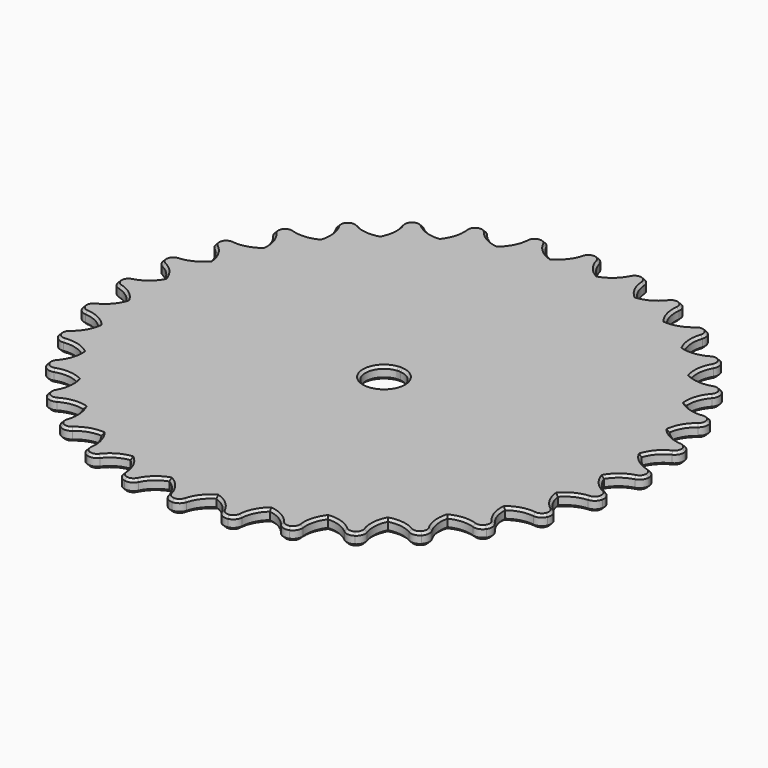
from build123d import *

# Parameters (mm, degrees)
F1_DEPTH    = 3.175
F2_C1_SIZE  = 0.635
F2_C2_SIZE  = 0.635
F2_C3_SIZE  = 0.635
F2_C4_SIZE  = 0.635
F2_C5_SIZE  = 0.635
F2_C6_SIZE  = 0.635
F2_C7_SIZE  = 0.635
F2_C8_SIZE  = 0.635
F2_C9_SIZE  = 0.635
F2_C10_SIZE = 0.635
F2_C11_SIZE = 0.635
F2_C12_SIZE = 0.635
F2_C13_SIZE = 0.635
F2_C14_SIZE = 0.635
F2_C15_SIZE = 0.635
F2_C16_SIZE = 0.635
F2_C17_SIZE = 0.635
F2_C18_SIZE = 0.635
F2_C19_SIZE = 0.635
F2_C20_SIZE = 0.635
F2_C21_SIZE = 0.635
F2_C22_SIZE = 0.635
F2_C23_SIZE = 0.635
F2_C24_SIZE = 0.635
F2_C25_SIZE = 0.635
F2_C26_SIZE = 0.635
F2_C27_SIZE = 0.635
F2_C28_SIZE = 0.635
F2_C29_SIZE = 0.635
F2_C30_SIZE = 0.635
F2_C31_SIZE = 0.635
F2_C32_SIZE = 0.635
F2_C33_SIZE = 0.635
F2_C34_SIZE = 0.635
F2_C35_SIZE = 0.635
F2_C36_SIZE = 0.635
F2_C37_SIZE = 0.635
F2_C38_SIZE = 0.635
F2_C39_SIZE = 0.635
F2_C40_SIZE = 0.635
F2_C41_SIZE = 0.635
F2_C42_SIZE = 0.635
F2_C43_SIZE = 0.635
F2_C44_SIZE = 0.635
F2_C45_SIZE = 0.635
F2_C46_SIZE = 0.635
F2_C47_SIZE = 0.635
F2_C48_SIZE = 0.635
F2_C49_SIZE = 0.635
F2_C50_SIZE = 0.635
F2_C51_SIZE = 0.635
F2_C52_SIZE = 0.635
F2_C53_SIZE = 0.635
F2_C54_SIZE = 0.635
F2_C55_SIZE = 0.635
F2_C56_SIZE = 0.635
F2_C57_SIZE = 0.635
F2_C58_SIZE = 0.635
F2_C59_SIZE = 0.635
F2_C60_SIZE = 0.635
F2_C61_SIZE = 0.635
F2_C62_SIZE = 0.635
F2_C63_SIZE = 0.635
F2_C64_SIZE = 0.635
F2_C65_SIZE = 0.635
F2_C66_SIZE = 0.635


with BuildPart() as f1:
    # F0 (on Top) → F1 (new body)
    with BuildSketch(Plane.XY):
        with BuildLine():
            ThreePointArc((66.1962592173, -2.3001108739), (67.4691190077, -1.4496131528), (67.9611963661, 0))
            ThreePointArc((67.9611963661, 0), (67.4691190077, 1.4496131528), (66.1962592173, 2.3001108739))
            ThreePointArc((66.1962592173, 2.3001108739), (63.3844227667, 3.6851664557), (61.3145216156, 6.0389532801))
            ThreePointArc((61.3145216156, 6.0389532801), (62.8854491669, 8.7513304327), (65.3730460291, 10.6583346386))
            ThreePointArc((65.3730460291, 10.6583346386), (66.4555243163, 11.7408129411), (66.6553410213, 13.25857175))
            ThreePointArc((66.6553410213, 13.25857175), (65.8899132823, 14.5843314182), (64.475587287, 15.1701644153))
            ThreePointArc((64.475587287, 15.1701644153), (61.4475685459, 15.980044464), (58.9582389354, 17.8847862524))
            ThreePointArc((58.9582389354, 17.8847862524), (59.9698230223, 20.8515186005), (62.0375833437, 23.2071863281))
            ThreePointArc((62.0375833437, 23.2071863281), (62.8880810643, 24.4800461171), (62.7879583288, 26.0076238902))
            ThreePointArc((62.7879583288, 26.0076238902), (61.7785951922, 27.1585819617), (60.2771546956, 27.4572370458))
            ThreePointArc((60.2771546956, 27.4572370458), (57.149318726, 27.6608183252), (54.3362241972, 29.0433169189))
            ThreePointArc((54.3362241972, 29.0433169189), (54.7495902103, 32.1503946021), (56.3180511214, 34.8641988618))
            ThreePointArc((56.3180511214, 34.8641988618), (56.9038841373, 36.2785248291), (56.5076696537, 37.7572176123))
            ThreePointArc((56.5076696537, 37.7572176123), (55.2931603573, 38.6891434377), (53.7623048531, 38.6891434549))
            ThreePointArc((53.7623048531, 38.6891434549), (50.6548526373, 38.2786024505), (47.6260988352, 39.0857292039))
            ThreePointArc((47.6260988352, 39.0857292039), (47.4253613505, 42.2137489692), (48.4342477781, 45.1813997853))
            ThreePointArc((48.4342477781, 45.1813997853), (48.7329028615, 46.6828402805), (48.055822808, 48.055822808))
            ThreePointArc((48.055822808, 48.055822808), (46.6828402805, 48.7329028615), (45.1813997853, 48.4342477781))
            ThreePointArc((45.1813997853, 48.4342477781), (42.2137489692, 47.4253613505), (39.0857292039, 47.6260988352))
            ThreePointArc((39.0857292039, 47.6260988352), (38.2786024505, 50.6548526373), (38.6891434549, 53.7623048531))
            ThreePointArc((38.6891434549, 53.7623048531), (38.6891434688, 55.2931602656), (37.7572177733, 56.5076695461))
            ThreePointArc((37.7572177733, 56.5076695461), (36.2785249257, 56.9038841436), (34.8641988618, 56.3180511214))
            ThreePointArc((34.8641988618, 56.3180511214), (32.1503946021, 54.7495902103), (29.0433169189, 54.3362241972))
            ThreePointArc((29.0433169189, 54.3362241972), (27.6608183252, 57.149318726), (27.4572370458, 60.2771546956))
            ThreePointArc((27.4572370458, 60.2771546956), (27.1585819525, 61.7785952082), (26.007623856, 62.7879583429))
            ThreePointArc((26.007623856, 62.7879583429), (24.4800460992, 62.8880810595), (23.2071863281, 62.0375833437))
            ThreePointArc((23.2071863281, 62.0375833437), (20.8515186005, 59.9698230223), (17.8847862524, 58.9582389354))
            ThreePointArc((17.8847862524, 58.9582389354), (15.980044464, 61.4475685459), (15.1701644153, 64.475587287))
            ThreePointArc((15.1701644153, 64.475587287), (14.5843314707, 65.8899132225), (13.2585719061, 66.6553409902))
            ThreePointArc((13.2585719061, 66.6553409902), (11.7408130125, 66.4555243514), (10.6583346386, 65.3730460291))
            ThreePointArc((10.6583346386, 65.3730460291), (8.7513304327, 62.8854491669), (6.0389532801, 61.3145216156))
            Line((6.0389532801, 61.3145216156), (0.4668066308, 4.7395672608))
            ThreePointArc((0.4668066308, 4.7395672608), (3.5287797345, 3.1982995225), (4.7625, 0))
            ThreePointArc((4.7625, 0), (-3.1982995225, -3.5287797345), (-0.4668066308, 4.7395672608))
            Line((-0.4668066308, 4.7395672608), (-6.0389532801, 61.3145216156))
            ThreePointArc((-6.0389532801, 61.3145216156), (-8.7513304327, 62.8854491669), (-10.6583346386, 65.3730460291))
            ThreePointArc((-10.6583346386, 65.3730460291), (-11.7408128353, 66.4555242641), (-13.2585715186, 66.6553410673))
            ThreePointArc((-13.2585715186, 66.6553410673), (-14.5843313404, 65.889913371), (-15.1701644153, 64.475587287))
            ThreePointArc((-15.1701644153, 64.475587287), (-15.980044464, 61.4475685459), (-17.8847862524, 58.9582389354))
            ThreePointArc((-17.8847862524, 58.9582389354), (-20.8515186005, 59.9698230223), (-23.2071863281, 62.0375833437))
            ThreePointArc((-23.2071863281, 62.0375833437), (-24.4800461298, 62.8880810677), (-26.0076239146, 62.7879583187))
            ThreePointArc((-26.0076239146, 62.7879583187), (-27.1585819683, 61.7785951807), (-27.4572370458, 60.2771546956))
            ThreePointArc((-27.4572370458, 60.2771546956), (-27.6608183252, 57.149318726), (-29.0433169189, 54.3362241972))
            ThreePointArc((-29.0433169189, 54.3362241972), (-32.1503946021, 54.7495902103), (-34.8641988618, 56.3180511214))
            ThreePointArc((-34.8641988618, 56.3180511214), (-36.278524843, 56.9038841382), (-37.7572176355, 56.5076696382))
            ThreePointArc((-37.7572176355, 56.5076696382), (-38.6891434422, 55.2931603441), (-38.6891434549, 53.7623048531))
            ThreePointArc((-38.6891434549, 53.7623048531), (-38.2786024505, 50.6548526373), (-39.0857292039, 47.6260988352))
            ThreePointArc((-39.0857292039, 47.6260988352), (-42.2137489692, 47.4253613505), (-45.1813997853, 48.4342477781))
            ThreePointArc((-45.1813997853, 48.4342477781), (-46.6828402805, 48.7329028615), (-48.055822808, 48.055822808))
            ThreePointArc((-48.055822808, 48.055822808), (-48.7329028615, 46.6828402805), (-48.4342477781, 45.1813997853))
            ThreePointArc((-48.4342477781, 45.1813997853), (-47.4253613505, 42.2137489692), (-47.6260988352, 39.0857292039))
            ThreePointArc((-47.6260988352, 39.0857292039), (-50.6548526373, 38.2786024505), (-53.7623048531, 38.6891434549))
            ThreePointArc((-53.7623048531, 38.6891434549), (-55.2931603441, 38.6891434422), (-56.5076696382, 37.7572176355))
            ThreePointArc((-56.5076696382, 37.7572176355), (-56.9038841382, 36.278524843), (-56.3180511214, 34.8641988618))
            ThreePointArc((-56.3180511214, 34.8641988618), (-54.7495902103, 32.1503946021), (-54.3362241972, 29.0433169189))
            ThreePointArc((-54.3362241972, 29.0433169189), (-57.149318726, 27.6608183252), (-60.2771546956, 27.4572370458))
            ThreePointArc((-60.2771546956, 27.4572370458), (-61.7785951621, 27.158581979), (-62.7879583023, 26.0076239542))
            ThreePointArc((-62.7879583023, 26.0076239542), (-62.8880810733, 24.4800461505), (-62.0375833437, 23.2071863281))
            ThreePointArc((-62.0375833437, 23.2071863281), (-59.9698230223, 20.8515186005), (-58.9582389354, 17.8847862524))
            ThreePointArc((-58.9582389354, 17.8847862524), (-61.4475685459, 15.980044464), (-64.475587287, 15.1701644153))
            ThreePointArc((-64.475587287, 15.1701644153), (-65.8899133548, 14.5843313546), (-66.6553410589, 13.2585715607))
            ThreePointArc((-66.6553410589, 13.2585715607), (-66.4555242736, 11.7408128546), (-65.3730460291, 10.6583346386))
            ThreePointArc((-65.3730460291, 10.6583346386), (-62.8854491669, 8.7513304327), (-61.3145216156, 6.0389532801))
            ThreePointArc((-61.3145216156, 6.0389532801), (-63.3844227667, 3.6851664557), (-66.1962592173, 2.3001108739))
            ThreePointArc((-66.1962592173, 2.3001108739), (-67.4691190077, 1.4496131528), (-67.9611963661, 0))
            ThreePointArc((-67.9611963661, 0), (-67.4691190077, -1.4496131528), (-66.1962592173, -2.3001108739))
            ThreePointArc((-66.1962592173, -2.3001108739), (-63.3844227667, -3.6851664557), (-61.3145216156, -6.0389532801))
            ThreePointArc((-61.3145216156, -6.0389532801), (-62.8854491669, -8.7513304327), (-65.3730460291, -10.6583346386))
            ThreePointArc((-65.3730460291, -10.6583346386), (-66.4555242713, -11.74081285), (-66.6553410609, -13.2585715508))
            ThreePointArc((-66.6553410609, -13.2585715508), (-65.8899133586, -14.5843313513), (-64.475587287, -15.1701644153))
            ThreePointArc((-64.475587287, -15.1701644153), (-61.4475685459, -15.980044464), (-58.9582389354, -17.8847862524))
            ThreePointArc((-58.9582389354, -17.8847862524), (-59.9698230223, -20.8515186005), (-62.0375833437, -23.2071863281))
            ThreePointArc((-62.0375833437, -23.2071863281), (-62.8880810643, -24.480046117), (-62.7879583288, -26.0076238901))
            ThreePointArc((-62.7879583288, -26.0076238901), (-61.7785951922, -27.1585819617), (-60.2771546956, -27.4572370458))
            ThreePointArc((-60.2771546956, -27.4572370458), (-57.149318726, -27.6608183252), (-54.3362241972, -29.0433169189))
            ThreePointArc((-54.3362241972, -29.0433169189), (-54.7495902103, -32.1503946021), (-56.3180511214, -34.8641988618))
            ThreePointArc((-56.3180511214, -34.8641988618), (-56.9038841382, -36.278524843), (-56.5076696382, -37.7572176355))
            ThreePointArc((-56.5076696382, -37.7572176355), (-55.2931603441, -38.6891434422), (-53.7623048531, -38.6891434549))
            ThreePointArc((-53.7623048531, -38.6891434549), (-50.6548526373, -38.2786024505), (-47.6260988352, -39.0857292039))
            ThreePointArc((-47.6260988352, -39.0857292039), (-47.4253613505, -42.2137489692), (-48.4342477781, -45.1813997853))
            ThreePointArc((-48.4342477781, -45.1813997853), (-48.7329028609, -46.6828402852), (-48.0558228014, -48.0558228147))
            ThreePointArc((-48.0558228014, -48.0558228147), (-46.6828402759, -48.7329028621), (-45.1813997853, -48.4342477781))
            ThreePointArc((-45.1813997853, -48.4342477781), (-42.2137489692, -47.4253613505), (-39.0857292039, -47.6260988352))
            ThreePointArc((-39.0857292039, -47.6260988352), (-38.2786024505, -50.6548526373), (-38.6891434549, -53.7623048531))
            ThreePointArc((-38.6891434549, -53.7623048531), (-38.6891434422, -55.2931603441), (-37.7572176355, -56.5076696382))
            ThreePointArc((-37.7572176355, -56.5076696382), (-36.278524843, -56.9038841382), (-34.8641988618, -56.3180511214))
            ThreePointArc((-34.8641988618, -56.3180511214), (-32.1503946021, -54.7495902103), (-29.0433169189, -54.3362241972))
            ThreePointArc((-29.0433169189, -54.3362241972), (-27.6608183252, -57.149318726), (-27.4572370458, -60.2771546956))
            ThreePointArc((-27.4572370458, -60.2771546956), (-27.158581979, -61.7785951621), (-26.0076239542, -62.7879583023))
            ThreePointArc((-26.0076239542, -62.7879583023), (-24.4800461505, -62.8880810733), (-23.2071863281, -62.0375833437))
            ThreePointArc((-23.2071863281, -62.0375833437), (-20.8515186005, -59.9698230223), (-17.8847862524, -58.9582389354))
            ThreePointArc((-17.8847862524, -58.9582389354), (-15.980044464, -61.4475685459), (-15.1701644153, -64.475587287))
            ThreePointArc((-15.1701644153, -64.475587287), (-14.5843314145, -65.8899132865), (-13.258571739, -66.6553410235))
            ThreePointArc((-13.258571739, -66.6553410235), (-11.7408129361, -66.4555243138), (-10.6583346386, -65.3730460291))
            ThreePointArc((-10.6583346386, -65.3730460291), (-8.7513304327, -62.8854491669), (-6.0389532801, -61.3145216156))
            ThreePointArc((-6.0389532801, -61.3145216156), (-3.6851664557, -63.3844227667), (-2.3001108739, -66.1962592173))
            ThreePointArc((-2.3001108739, -66.1962592173), (-1.4496131528, -67.4691190077), (0, -67.9611963661))
            ThreePointArc((0, -67.9611963661), (1.4496131528, -67.4691190077), (2.3001108739, -66.1962592173))
            ThreePointArc((2.3001108739, -66.1962592173), (3.6851664557, -63.3844227667), (6.0389532801, -61.3145216156))
            ThreePointArc((6.0389532801, -61.3145216156), (8.7513304327, -62.8854491669), (10.6583346386, -65.3730460291))
            ThreePointArc((10.6583346386, -65.3730460291), (11.7408129169, -66.4555243043), (13.258571697, -66.6553410318))
            ThreePointArc((13.258571697, -66.6553410318), (14.5843314004, -65.8899133026), (15.1701644153, -64.475587287))
            ThreePointArc((15.1701644153, -64.475587287), (15.980044464, -61.4475685459), (17.8847862524, -58.9582389354))
            ThreePointArc((17.8847862524, -58.9582389354), (20.8515186005, -59.9698230223), (23.2071863281, -62.0375833437))
            ThreePointArc((23.2071863281, -62.0375833437), (24.4800461505, -62.8880810733), (26.0076239542, -62.7879583023))
            ThreePointArc((26.0076239542, -62.7879583023), (27.158581979, -61.7785951621), (27.4572370458, -60.2771546956))
            ThreePointArc((27.4572370458, -60.2771546956), (27.6608183252, -57.149318726), (29.0433169189, -54.3362241972))
            ThreePointArc((29.0433169189, -54.3362241972), (32.1503946021, -54.7495902103), (34.8641988618, -56.3180511214))
            ThreePointArc((34.8641988618, -56.3180511214), (36.278524843, -56.9038841382), (37.7572176355, -56.5076696382))
            ThreePointArc((37.7572176355, -56.5076696382), (38.6891434422, -55.2931603441), (38.6891434549, -53.7623048531))
            ThreePointArc((38.6891434549, -53.7623048531), (38.2786024505, -50.6548526373), (39.0857292039, -47.6260988352))
            ThreePointArc((39.0857292039, -47.6260988352), (42.2137489692, -47.4253613505), (45.1813997853, -48.4342477781))
            ThreePointArc((45.1813997853, -48.4342477781), (46.6828402846, -48.7329028609), (48.0558228138, -48.0558228022))
            ThreePointArc((48.0558228138, -48.0558228022), (48.732902862, -46.6828402765), (48.4342477781, -45.1813997853))
            ThreePointArc((48.4342477781, -45.1813997853), (47.4253613505, -42.2137489692), (47.6260988352, -39.0857292039))
            ThreePointArc((47.6260988352, -39.0857292039), (50.6548526373, -38.2786024505), (53.7623048531, -38.6891434549))
            ThreePointArc((53.7623048531, -38.6891434549), (55.2931603441, -38.6891434422), (56.5076696382, -37.7572176355))
            ThreePointArc((56.5076696382, -37.7572176355), (56.9038841382, -36.278524843), (56.3180511214, -34.8641988618))
            ThreePointArc((56.3180511214, -34.8641988618), (54.7495902103, -32.1503946021), (54.3362241972, -29.0433169189))
            ThreePointArc((54.3362241972, -29.0433169189), (57.149318726, -27.6608183252), (60.2771546956, -27.4572370458))
            ThreePointArc((60.2771546956, -27.4572370458), (61.7785951621, -27.158581979), (62.7879583023, -26.0076239542))
            ThreePointArc((62.7879583023, -26.0076239542), (62.8880810733, -24.4800461505), (62.0375833437, -23.2071863281))
            ThreePointArc((62.0375833437, -23.2071863281), (59.9698230223, -20.8515186005), (58.9582389354, -17.8847862524))
            ThreePointArc((58.9582389354, -17.8847862524), (61.4475685459, -15.980044464), (64.475587287, -15.1701644153))
            ThreePointArc((64.475587287, -15.1701644153), (65.8899133026, -14.5843314004), (66.6553410318, -13.258571697))
            ThreePointArc((66.6553410318, -13.258571697), (66.4555243043, -11.7408129169), (65.3730460291, -10.6583346386))
            ThreePointArc((65.3730460291, -10.6583346386), (62.8854491669, -8.7513304327), (61.3145216156, -6.0389532801))
            ThreePointArc((61.3145216156, -6.0389532801), (63.3844227667, -3.6851664557), (66.1962592173, -2.3001108739))
        make_face()
        with BuildLine():
            Line((0.4668066308, 4.7395672608), (6.0389532801, 61.3145216156))
            ThreePointArc((6.0389532801, 61.3145216156), (3.6851664557, 63.3844227667), (2.3001108739, 66.1962592173))
            Line((2.3001108739, 66.1962592173), (1.190625, 65.8989733733))
            ThreePointArc((1.190625, 65.8989733733), (0.6163128512, 65.6610854923), (0, 65.5799463661))
            Line((0, 65.5799463661), (0, 4.7625))
            ThreePointArc((0, 4.7625), (0.233684799, 4.7567633602), (0.4668066308, 4.7395672608))
        make_face()
        with BuildLine():
            Line((0, 4.7625), (0, 65.5799463661))
            ThreePointArc((0, 65.5799463661), (-0.6163128512, 65.6610854923), (-1.190625, 65.8989733733))
            Line((-1.190625, 65.8989733733), (-2.3001108739, 66.1962592173))
            ThreePointArc((-2.3001108739, 66.1962592173), (-3.6851664557, 63.3844227667), (-6.0389532801, 61.3145216156))
            Line((-6.0389532801, 61.3145216156), (-0.4668066308, 4.7395672608))
            ThreePointArc((-0.4668066308, 4.7395672608), (-0.233684799, 4.7567633602), (0, 4.7625))
        make_face()
        with BuildLine():
            ThreePointArc((2.0622229928, 66.7705713661), (1.190625, 67.6421693589), (0, 67.9611963661))
            Line((0, 67.9611963661), (0, 65.5799463661))
            Line((0, 65.5799463661), (1.190625, 65.8989733733))
            ThreePointArc((1.190625, 65.8989733733), (1.6837980227, 66.2773983434), (2.0622229928, 66.7705713661))
        make_face()
        with BuildLine():
            ThreePointArc((2.3001108739, 66.1962592173), (2.1999881368, 66.4912112894), (2.0622229928, 66.7705713661))
            ThreePointArc((2.0622229928, 66.7705713661), (1.6837980227, 66.2773983434), (1.190625, 65.8989733733))
            Line((1.190625, 65.8989733733), (2.3001108739, 66.1962592173))
        make_face()
        with BuildLine():
            Line((1.190625, 65.8989733733), (0, 65.5799463661))
            ThreePointArc((0, 65.5799463661), (0.6163128512, 65.6610854923), (1.190625, 65.8989733733))
        make_face()
        with BuildLine():
            ThreePointArc((-1.190625, 65.8989733733), (-0.6163128512, 65.6610854923), (0, 65.5799463661))
            Line((0, 65.5799463661), (-1.190625, 65.8989733733))
        make_face()
        with BuildLine():
            Line((0, 65.5799463661), (0, 67.9611963661))
            ThreePointArc((0, 67.9611963661), (-1.190625, 67.6421693589), (-2.0622229928, 66.7705713661))
            ThreePointArc((-2.0622229928, 66.7705713661), (-1.6837980227, 66.2773983434), (-1.190625, 65.8989733733))
            Line((-1.190625, 65.8989733733), (0, 65.5799463661))
        make_face()
        with BuildLine():
            ThreePointArc((-1.190625, 65.8989733733), (-1.6837980227, 66.2773983434), (-2.0622229928, 66.7705713661))
            ThreePointArc((-2.0622229928, 66.7705713661), (-2.1999881368, 66.4912112894), (-2.3001108739, 66.1962592173))
            Line((-2.3001108739, 66.1962592173), (-1.190625, 65.8989733733))
        make_face()
    extrude(amount=F1_DEPTH)

    # F2: chamfer of 0.635 on 194 edges, made by hand

    # F2_c1
    f2_c1_edges = [f1.edges().sort_by_distance(p)[0] for p in [
        (-3.6851664557, 63.3844227667, 0),
        (3.6851664557, 63.3844227667, 0),
        (0, 67.9611963661, 0),
    ]]
    chamfer(f2_c1_edges, length=F2_C1_SIZE)

    # F2_c2
    f2_c2_edges = [f1.edges().sort_by_distance(p)[0] for p in [
        (-3.6851664557, 63.3844227667, 3.175),
        (3.6851664557, 63.3844227667, 3.175),
        (0, 67.9611963661, 3.175),
    ]]
    chamfer(f2_c2_edges, length=F2_C2_SIZE)

    # F2_c3
    f2_c3_edges = [f1.edges().sort_by_distance(p)[0] for p in [
        (-8.7513304327, 62.8854491669, 0),
        (-13.2585716837, 66.6553410345, 0),
        (-15.980044464, 61.4475685459, 0),
    ]]
    chamfer(f2_c3_edges, length=F2_C3_SIZE)

    # F2_c4
    f2_c4_edges = [f1.edges().sort_by_distance(p)[0] for p in [
        (-8.7513304327, 62.8854491669, 3.175),
        (-13.2585716837, 66.6553410345, 3.175),
        (-15.980044464, 61.4475685459, 3.175),
    ]]
    chamfer(f2_c4_edges, length=F2_C4_SIZE)

    # F2_c5
    f2_c5_edges = [f1.edges().sort_by_distance(p)[0] for p in [
        (-20.8515186005, 59.9698230223, 0),
        (-26.007623893, 62.7879583276, 0),
        (-27.6608183252, 57.149318726, 0),
    ]]
    chamfer(f2_c5_edges, length=F2_C5_SIZE)

    # F2_c6
    f2_c6_edges = [f1.edges().sort_by_distance(p)[0] for p in [
        (-20.8515186005, 59.9698230223, 3.175),
        (-26.007623893, 62.7879583276, 3.175),
        (-27.6608183252, 57.149318726, 3.175),
    ]]
    chamfer(f2_c6_edges, length=F2_C6_SIZE)

    # F2_c7
    f2_c7_edges = [f1.edges().sort_by_distance(p)[0] for p in [
        (-32.1503946021, 54.7495902103, 0),
        (-37.7572177014, 56.5076695941, 0),
        (-38.2786024505, 50.6548526373, 0),
    ]]
    chamfer(f2_c7_edges, length=F2_C7_SIZE)

    # F2_c8
    f2_c8_edges = [f1.edges().sort_by_distance(p)[0] for p in [
        (-32.1503946021, 54.7495902103, 3.175),
        (-37.7572177014, 56.5076695941, 3.175),
        (-38.2786024505, 50.6548526373, 3.175),
    ]]
    chamfer(f2_c8_edges, length=F2_C8_SIZE)

    # F2_c9
    f2_c9_edges = [f1.edges().sort_by_distance(p)[0] for p in [
        (-42.2137489692, 47.4253613505, 0),
        (-48.055822808, 48.055822808, 0),
        (-47.4253613505, 42.2137489692, 0),
    ]]
    chamfer(f2_c9_edges, length=F2_C9_SIZE)

    # F2_c10
    f2_c10_edges = [f1.edges().sort_by_distance(p)[0] for p in [
        (-42.2137489692, 47.4253613505, 3.175),
        (-48.055822808, 48.055822808, 3.175),
        (-47.4253613505, 42.2137489692, 3.175),
    ]]
    chamfer(f2_c10_edges, length=F2_C10_SIZE)

    # F2_c11
    f2_c11_edges = [f1.edges().sort_by_distance(p)[0] for p in [
        (-50.6548526373, 38.2786024505, 0),
        (-56.5076695941, 37.7572177014, 0),
        (-54.7495902103, 32.1503946021, 0),
    ]]
    chamfer(f2_c11_edges, length=F2_C11_SIZE)

    # F2_c12
    f2_c12_edges = [f1.edges().sort_by_distance(p)[0] for p in [
        (-50.6548526373, 38.2786024505, 3.175),
        (-56.5076695941, 37.7572177014, 3.175),
        (-54.7495902103, 32.1503946021, 3.175),
    ]]
    chamfer(f2_c12_edges, length=F2_C12_SIZE)

    # F2_c13
    f2_c13_edges = [f1.edges().sort_by_distance(p)[0] for p in [
        (-57.149318726, 27.6608183252, 0),
        (-62.7879583276, 26.007623893, 0),
        (-59.9698230223, 20.8515186005, 0),
    ]]
    chamfer(f2_c13_edges, length=F2_C13_SIZE)

    # F2_c14
    f2_c14_edges = [f1.edges().sort_by_distance(p)[0] for p in [
        (-57.149318726, 27.6608183252, 3.175),
        (-62.7879583276, 26.007623893, 3.175),
        (-59.9698230223, 20.8515186005, 3.175),
    ]]
    chamfer(f2_c14_edges, length=F2_C14_SIZE)

    # F2_c15
    f2_c15_edges = [f1.edges().sort_by_distance(p)[0] for p in [
        (-61.4475685459, 15.980044464, 0),
        (-66.6553410345, 13.2585716837, 0),
        (-62.8854491669, 8.7513304327, 0),
    ]]
    chamfer(f2_c15_edges, length=F2_C15_SIZE)

    # F2_c16
    f2_c16_edges = [f1.edges().sort_by_distance(p)[0] for p in [
        (-61.4475685459, 15.980044464, 3.175),
        (-66.6553410345, 13.2585716837, 3.175),
        (-62.8854491669, 8.7513304327, 3.175),
    ]]
    chamfer(f2_c16_edges, length=F2_C16_SIZE)

    # F2_c17
    f2_c17_edges = [f1.edges().sort_by_distance(p)[0] for p in [
        (-63.3844227667, 3.6851664557, 0),
        (-67.9611963661, 0, 0),
        (-63.3844227667, -3.6851664557, 0),
    ]]
    chamfer(f2_c17_edges, length=F2_C17_SIZE)

    # F2_c18
    f2_c18_edges = [f1.edges().sort_by_distance(p)[0] for p in [
        (-63.3844227667, 3.6851664557, 3.175),
        (-67.9611963661, 0, 3.175),
        (-63.3844227667, -3.6851664557, 3.175),
    ]]
    chamfer(f2_c18_edges, length=F2_C18_SIZE)

    # F2_c19
    f2_c19_edges = [f1.edges().sort_by_distance(p)[0] for p in [
        (-62.8854491669, -8.7513304327, 0),
        (-66.6553410345, -13.2585716837, 0),
        (-61.4475685459, -15.980044464, 0),
    ]]
    chamfer(f2_c19_edges, length=F2_C19_SIZE)

    # F2_c20
    f2_c20_edges = [f1.edges().sort_by_distance(p)[0] for p in [
        (-62.8854491669, -8.7513304327, 3.175),
        (-66.6553410345, -13.2585716837, 3.175),
        (-61.4475685459, -15.980044464, 3.175),
    ]]
    chamfer(f2_c20_edges, length=F2_C20_SIZE)

    # F2_c21
    f2_c21_edges = [f1.edges().sort_by_distance(p)[0] for p in [
        (-59.9698230223, -20.8515186005, 0),
        (-62.7879583276, -26.007623893, 0),
        (-57.149318726, -27.6608183252, 0),
    ]]
    chamfer(f2_c21_edges, length=F2_C21_SIZE)

    # F2_c22
    f2_c22_edges = [f1.edges().sort_by_distance(p)[0] for p in [
        (-59.9698230223, -20.8515186005, 3.175),
        (-62.7879583276, -26.007623893, 3.175),
        (-57.149318726, -27.6608183252, 3.175),
    ]]
    chamfer(f2_c22_edges, length=F2_C22_SIZE)

    # F2_c23
    f2_c23_edges = [f1.edges().sort_by_distance(p)[0] for p in [
        (-54.7495902103, -32.1503946021, 0),
        (-56.5076695941, -37.7572177014, 0),
        (-50.6548526373, -38.2786024505, 0),
    ]]
    chamfer(f2_c23_edges, length=F2_C23_SIZE)

    # F2_c24
    f2_c24_edges = [f1.edges().sort_by_distance(p)[0] for p in [
        (-54.7495902103, -32.1503946021, 3.175),
        (-56.5076695941, -37.7572177014, 3.175),
        (-50.6548526373, -38.2786024505, 3.175),
    ]]
    chamfer(f2_c24_edges, length=F2_C24_SIZE)

    # F2_c25
    f2_c25_edges = [f1.edges().sort_by_distance(p)[0] for p in [
        (-47.4253613505, -42.2137489692, 0),
        (-48.055822808, -48.055822808, 0),
        (-42.2137489692, -47.4253613505, 0),
    ]]
    chamfer(f2_c25_edges, length=F2_C25_SIZE)

    # F2_c26
    f2_c26_edges = [f1.edges().sort_by_distance(p)[0] for p in [
        (-47.4253613505, -42.2137489692, 3.175),
        (-48.055822808, -48.055822808, 3.175),
        (-42.2137489692, -47.4253613505, 3.175),
    ]]
    chamfer(f2_c26_edges, length=F2_C26_SIZE)

    # F2_c27
    f2_c27_edges = [f1.edges().sort_by_distance(p)[0] for p in [
        (-38.2786024505, -50.6548526373, 0),
        (-37.7572177014, -56.5076695941, 0),
        (-32.1503946021, -54.7495902103, 0),
    ]]
    chamfer(f2_c27_edges, length=F2_C27_SIZE)

    # F2_c28
    f2_c28_edges = [f1.edges().sort_by_distance(p)[0] for p in [
        (-38.2786024505, -50.6548526373, 3.175),
        (-37.7572177014, -56.5076695941, 3.175),
        (-32.1503946021, -54.7495902103, 3.175),
    ]]
    chamfer(f2_c28_edges, length=F2_C28_SIZE)

    # F2_c29
    f2_c29_edges = [f1.edges().sort_by_distance(p)[0] for p in [
        (-27.6608183252, -57.149318726, 0),
        (-26.007623893, -62.7879583276, 0),
        (-20.8515186005, -59.9698230223, 0),
    ]]
    chamfer(f2_c29_edges, length=F2_C29_SIZE)

    # F2_c30
    f2_c30_edges = [f1.edges().sort_by_distance(p)[0] for p in [
        (-27.6608183252, -57.149318726, 3.175),
        (-26.007623893, -62.7879583276, 3.175),
        (-20.8515186005, -59.9698230223, 3.175),
    ]]
    chamfer(f2_c30_edges, length=F2_C30_SIZE)

    # F2_c31
    f2_c31_edges = [f1.edges().sort_by_distance(p)[0] for p in [
        (-15.980044464, -61.4475685459, 0),
        (-13.2585716837, -66.6553410345, 0),
        (-8.7513304327, -62.8854491669, 0),
    ]]
    chamfer(f2_c31_edges, length=F2_C31_SIZE)

    # F2_c32
    f2_c32_edges = [f1.edges().sort_by_distance(p)[0] for p in [
        (-15.980044464, -61.4475685459, 3.175),
        (-13.2585716837, -66.6553410345, 3.175),
        (-8.7513304327, -62.8854491669, 3.175),
    ]]
    chamfer(f2_c32_edges, length=F2_C32_SIZE)

    # F2_c33
    f2_c33_edges = [f1.edges().sort_by_distance(p)[0] for p in [
        (-3.6851664557, -63.3844227667, 0),
        (0, -67.9611963661, 0),
        (3.6851664557, -63.3844227667, 0),
    ]]
    chamfer(f2_c33_edges, length=F2_C33_SIZE)

    # F2_c34
    f2_c34_edges = [f1.edges().sort_by_distance(p)[0] for p in [
        (-3.6851664557, -63.3844227667, 3.175),
        (0, -67.9611963661, 3.175),
        (3.6851664557, -63.3844227667, 3.175),
    ]]
    chamfer(f2_c34_edges, length=F2_C34_SIZE)

    # F2_c35
    f2_c35_edges = [f1.edges().sort_by_distance(p)[0] for p in [
        (8.7513304327, -62.8854491669, 0),
        (13.2585716837, -66.6553410345, 0),
        (15.980044464, -61.4475685459, 0),
    ]]
    chamfer(f2_c35_edges, length=F2_C35_SIZE)

    # F2_c36
    f2_c36_edges = [f1.edges().sort_by_distance(p)[0] for p in [
        (8.7513304327, -62.8854491669, 3.175),
        (13.2585716837, -66.6553410345, 3.175),
        (15.980044464, -61.4475685459, 3.175),
    ]]
    chamfer(f2_c36_edges, length=F2_C36_SIZE)

    # F2_c37
    f2_c37_edges = [f1.edges().sort_by_distance(p)[0] for p in [
        (20.8515186005, -59.9698230223, 0),
        (26.007623893, -62.7879583276, 0),
        (27.6608183252, -57.149318726, 0),
    ]]
    chamfer(f2_c37_edges, length=F2_C37_SIZE)

    # F2_c38
    f2_c38_edges = [f1.edges().sort_by_distance(p)[0] for p in [
        (20.8515186005, -59.9698230223, 3.175),
        (26.007623893, -62.7879583276, 3.175),
        (27.6608183252, -57.149318726, 3.175),
    ]]
    chamfer(f2_c38_edges, length=F2_C38_SIZE)

    # F2_c39
    f2_c39_edges = [f1.edges().sort_by_distance(p)[0] for p in [
        (32.1503946021, -54.7495902103, 0),
        (37.7572177014, -56.5076695941, 0),
        (38.2786024505, -50.6548526373, 0),
    ]]
    chamfer(f2_c39_edges, length=F2_C39_SIZE)

    # F2_c40
    f2_c40_edges = [f1.edges().sort_by_distance(p)[0] for p in [
        (32.1503946021, -54.7495902103, 3.175),
        (37.7572177014, -56.5076695941, 3.175),
        (38.2786024505, -50.6548526373, 3.175),
    ]]
    chamfer(f2_c40_edges, length=F2_C40_SIZE)

    # F2_c41
    f2_c41_edges = [f1.edges().sort_by_distance(p)[0] for p in [
        (42.2137489692, -47.4253613505, 0),
        (48.055822808, -48.055822808, 0),
        (47.4253613505, -42.2137489692, 0),
    ]]
    chamfer(f2_c41_edges, length=F2_C41_SIZE)

    # F2_c42
    f2_c42_edges = [f1.edges().sort_by_distance(p)[0] for p in [
        (42.2137489692, -47.4253613505, 3.175),
        (48.055822808, -48.055822808, 3.175),
        (47.4253613505, -42.2137489692, 3.175),
    ]]
    chamfer(f2_c42_edges, length=F2_C42_SIZE)

    # F2_c43
    f2_c43_edges = [f1.edges().sort_by_distance(p)[0] for p in [
        (50.6548526373, -38.2786024505, 0),
        (56.5076695941, -37.7572177014, 0),
        (54.7495902103, -32.1503946021, 0),
    ]]
    chamfer(f2_c43_edges, length=F2_C43_SIZE)

    # F2_c44
    f2_c44_edges = [f1.edges().sort_by_distance(p)[0] for p in [
        (50.6548526373, -38.2786024505, 3.175),
        (56.5076695941, -37.7572177014, 3.175),
        (54.7495902103, -32.1503946021, 3.175),
    ]]
    chamfer(f2_c44_edges, length=F2_C44_SIZE)

    # F2_c45
    f2_c45_edges = [f1.edges().sort_by_distance(p)[0] for p in [
        (57.149318726, -27.6608183252, 0),
        (62.7879583276, -26.007623893, 0),
        (59.9698230223, -20.8515186005, 0),
    ]]
    chamfer(f2_c45_edges, length=F2_C45_SIZE)

    # F2_c46
    f2_c46_edges = [f1.edges().sort_by_distance(p)[0] for p in [
        (57.149318726, -27.6608183252, 3.175),
        (62.7879583276, -26.007623893, 3.175),
        (59.9698230223, -20.8515186005, 3.175),
    ]]
    chamfer(f2_c46_edges, length=F2_C46_SIZE)

    # F2_c47
    f2_c47_edges = [f1.edges().sort_by_distance(p)[0] for p in [
        (61.4475685459, -15.980044464, 0),
        (66.6553410345, -13.2585716837, 0),
        (62.8854491669, -8.7513304327, 0),
    ]]
    chamfer(f2_c47_edges, length=F2_C47_SIZE)

    # F2_c48
    f2_c48_edges = [f1.edges().sort_by_distance(p)[0] for p in [
        (61.4475685459, -15.980044464, 3.175),
        (66.6553410345, -13.2585716837, 3.175),
        (62.8854491669, -8.7513304327, 3.175),
    ]]
    chamfer(f2_c48_edges, length=F2_C48_SIZE)

    # F2_c49
    f2_c49_edges = [f1.edges().sort_by_distance(p)[0] for p in [
        (63.3844227667, -3.6851664557, 0),
        (67.9611963661, 0, 0),
        (63.3844227667, 3.6851664557, 0),
    ]]
    chamfer(f2_c49_edges, length=F2_C49_SIZE)

    # F2_c50
    f2_c50_edges = [f1.edges().sort_by_distance(p)[0] for p in [
        (63.3844227667, -3.6851664557, 3.175),
        (67.9611963661, 0, 3.175),
        (63.3844227667, 3.6851664557, 3.175),
    ]]
    chamfer(f2_c50_edges, length=F2_C50_SIZE)

    # F2_c51
    f2_c51_edges = [f1.edges().sort_by_distance(p)[0] for p in [
        (62.8854491669, 8.7513304327, 0),
        (66.6553410345, 13.2585716837, 0),
        (61.4475685459, 15.980044464, 0),
    ]]
    chamfer(f2_c51_edges, length=F2_C51_SIZE)

    # F2_c52
    f2_c52_edges = [f1.edges().sort_by_distance(p)[0] for p in [
        (62.8854491669, 8.7513304327, 3.175),
        (66.6553410345, 13.2585716837, 3.175),
        (61.4475685459, 15.980044464, 3.175),
    ]]
    chamfer(f2_c52_edges, length=F2_C52_SIZE)

    # F2_c53
    f2_c53_edges = [f1.edges().sort_by_distance(p)[0] for p in [
        (59.9698230223, 20.8515186005, 0),
        (62.7879583276, 26.007623893, 0),
        (57.149318726, 27.6608183252, 0),
    ]]
    chamfer(f2_c53_edges, length=F2_C53_SIZE)

    # F2_c54
    f2_c54_edges = [f1.edges().sort_by_distance(p)[0] for p in [
        (59.9698230223, 20.8515186005, 3.175),
        (62.7879583276, 26.007623893, 3.175),
        (57.149318726, 27.6608183252, 3.175),
    ]]
    chamfer(f2_c54_edges, length=F2_C54_SIZE)

    # F2_c55
    f2_c55_edges = [f1.edges().sort_by_distance(p)[0] for p in [
        (54.7495902103, 32.1503946021, 0),
        (56.5076695941, 37.7572177014, 0),
        (50.6548526373, 38.2786024505, 0),
    ]]
    chamfer(f2_c55_edges, length=F2_C55_SIZE)

    # F2_c56
    f2_c56_edges = [f1.edges().sort_by_distance(p)[0] for p in [
        (54.7495902103, 32.1503946021, 3.175),
        (56.5076695941, 37.7572177014, 3.175),
        (50.6548526373, 38.2786024505, 3.175),
    ]]
    chamfer(f2_c56_edges, length=F2_C56_SIZE)

    # F2_c57
    f2_c57_edges = [f1.edges().sort_by_distance(p)[0] for p in [
        (47.4253613505, 42.2137489692, 0),
        (48.055822808, 48.055822808, 0),
        (42.2137489692, 47.4253613505, 0),
    ]]
    chamfer(f2_c57_edges, length=F2_C57_SIZE)

    # F2_c58
    f2_c58_edges = [f1.edges().sort_by_distance(p)[0] for p in [
        (47.4253613505, 42.2137489692, 3.175),
        (48.055822808, 48.055822808, 3.175),
        (42.2137489692, 47.4253613505, 3.175),
    ]]
    chamfer(f2_c58_edges, length=F2_C58_SIZE)

    # F2_c59
    f2_c59_edges = [f1.edges().sort_by_distance(p)[0] for p in [
        (38.2786024505, 50.6548526373, 0),
        (37.7572177014, 56.5076695941, 0),
        (32.1503946021, 54.7495902103, 0),
    ]]
    chamfer(f2_c59_edges, length=F2_C59_SIZE)

    # F2_c60
    f2_c60_edges = [f1.edges().sort_by_distance(p)[0] for p in [
        (38.2786024505, 50.6548526373, 3.175),
        (37.7572177014, 56.5076695941, 3.175),
        (32.1503946021, 54.7495902103, 3.175),
    ]]
    chamfer(f2_c60_edges, length=F2_C60_SIZE)

    # F2_c61
    f2_c61_edges = [f1.edges().sort_by_distance(p)[0] for p in [
        (27.6608183252, 57.149318726, 0),
        (26.007623893, 62.7879583276, 0),
        (20.8515186005, 59.9698230223, 0),
    ]]
    chamfer(f2_c61_edges, length=F2_C61_SIZE)

    # F2_c62
    f2_c62_edges = [f1.edges().sort_by_distance(p)[0] for p in [
        (27.6608183252, 57.149318726, 3.175),
        (26.007623893, 62.7879583276, 3.175),
        (20.8515186005, 59.9698230223, 3.175),
    ]]
    chamfer(f2_c62_edges, length=F2_C62_SIZE)

    # F2_c63
    f2_c63_edges = [f1.edges().sort_by_distance(p)[0] for p in [
        (15.980044464, 61.4475685459, 0),
        (13.2585716837, 66.6553410345, 0),
        (8.7513304327, 62.8854491669, 0),
    ]]
    chamfer(f2_c63_edges, length=F2_C63_SIZE)

    # F2_c64
    f2_c64_edges = [f1.edges().sort_by_distance(p)[0] for p in [
        (15.980044464, 61.4475685459, 3.175),
        (13.2585716837, 66.6553410345, 3.175),
        (8.7513304327, 62.8854491669, 3.175),
    ]]
    chamfer(f2_c64_edges, length=F2_C64_SIZE)

    # F2_c65
    f2_c65_edges = [f1.edges().sort_by_distance(p)[0] for p in [
        (0.4668066308, -4.7395672608, 0),
    ]]
    chamfer(f2_c65_edges, length=F2_C65_SIZE)

    # F2_c66
    f2_c66_edges = [f1.edges().sort_by_distance(p)[0] for p in [
        (0.4668066308, -4.7395672608, 3.175),
    ]]
    chamfer(f2_c66_edges, length=F2_C66_SIZE)


solid = f1.part
